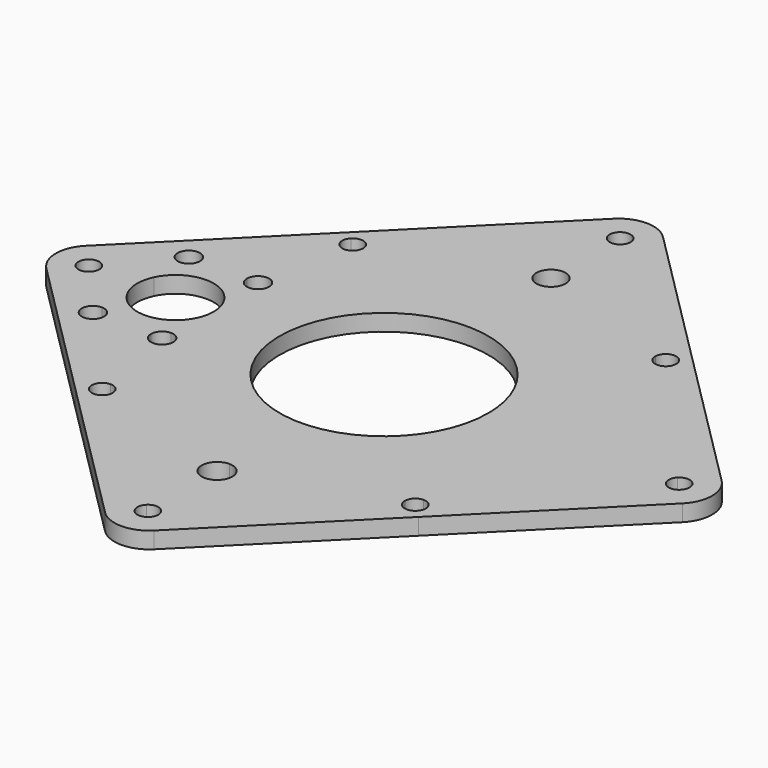
from build123d import *

# Parameters (mm, degrees)
F1_DEPTH = 2.38125
F2_R     = 5
F4_DEPTH = 25
F6_DEPTH = 25


# Not quite as in the source:
# - a feature names something its author has since deleted; it is built from what else it names


with BuildPart() as f1:
    # F0 (on Top) → F1 (new body)
    with BuildSketch(Plane.XY):
        with BuildLine():
            Line((19.9264068712, 22.5), (21.2132034356, 21.2132034356))
            Line((21.2132034356, 21.2132034356), (22.5, 19.9264068712))
            Line((22.5, 19.9264068712), (22.5, 21))
            ThreePointArc((22.5, 21), (21.4393398282, 21.4393398282), (21, 22.5))
            Line((21, 22.5), (19.9264068712, 22.5))
        make_face()
        with BuildLine():
            Line((-41.3657466994, 1.0606601718), (-22.5, 19.9264068712))
            Line((-22.5, 19.9264068712), (-22.5, 21))
            ThreePointArc((-22.5, 21), (-23.8858192988, 21.9259748515), (-23.5606601718, 23.5606601718))
            Line((-23.5606601718, 23.5606601718), (-24.6213203436, 24.6213203436))
            Line((-24.6213203436, 24.6213203436), (-49.2426406871, 0))
            Line((-49.2426406871, 0), (-24.6213203436, -24.6213203436))
            Line((-24.6213203436, -24.6213203436), (-23.5606601718, -23.5606601718))
            ThreePointArc((-23.5606601718, -23.5606601718), (-23.8858192988, -21.9259748515), (-22.5, -21))
            Line((-22.5, -21), (-22.5, -19.9264068712))
            Line((-22.5, -19.9264068712), (-41.3657466994, -1.0606601718))
            ThreePointArc((-41.3657466994, -1.0606601718), (-43.9264068712, 0), (-41.3657466994, 1.0606601718))
        make_face()
        with BuildLine():
            Line((21, -22.5), (19.9264068712, -22.5))
            Line((19.9264068712, -22.5), (1.0606601718, -41.3657466994))
            ThreePointArc((1.0606601718, -41.3657466994), (1.3858192988, -41.8523817226), (1.5, -42.4264068712))
            ThreePointArc((1.5, -42.4264068712), (-0.5740251485, -43.81222617), (-1.0606601718, -41.3657466994))
            Line((-1.0606601718, -41.3657466994), (-19.9264068712, -22.5))
            Line((-19.9264068712, -22.5), (-21, -22.5))
            ThreePointArc((-21, -22.5), (-21.9259748515, -23.8858192988), (-23.5606601718, -23.5606601718))
            Line((-23.5606601718, -23.5606601718), (-24.6213203436, -24.6213203436))
            Line((-24.6213203436, -24.6213203436), (0, -49.2426406871))
            Line((0, -49.2426406871), (24.6213203436, -24.6213203436))
            Line((24.6213203436, -24.6213203436), (23.5606601718, -23.5606601718))
            ThreePointArc((23.5606601718, -23.5606601718), (21.9259748515, -23.8858192988), (21, -22.5))
        make_face()
        with BuildLine():
            Line((22.5, 21), (22.5, 19.9264068712))
            Line((22.5, 19.9264068712), (41.3657466994, 1.0606601718))
            ThreePointArc((41.3657466994, 1.0606601718), (43.0004320197, 1.3858192988), (43.9264068712, 0))
            ThreePointArc((43.9264068712, 0), (43.0004320197, -1.3858192988), (41.3657466994, -1.0606601718))
            Line((41.3657466994, -1.0606601718), (22.5, -19.9264068712))
            Line((22.5, -19.9264068712), (22.5, -21))
            ThreePointArc((22.5, -21), (23.5606601718, -21.4393398282), (24, -22.5))
            ThreePointArc((24, -22.5), (23.8858192988, -23.0740251485), (23.5606601718, -23.5606601718))
            Line((23.5606601718, -23.5606601718), (24.6213203436, -24.6213203436))
            Line((24.6213203436, -24.6213203436), (49.2426406871, 0))
            Line((49.2426406871, 0), (0, 49.2426406871))
            Line((0, 49.2426406871), (-24.6213203436, 24.6213203436))
            Line((-24.6213203436, 24.6213203436), (-23.5606601718, 23.5606601718))
            ThreePointArc((-23.5606601718, 23.5606601718), (-21.9259748515, 23.8858192988), (-21, 22.5))
            Line((-21, 22.5), (-19.9264068712, 22.5))
            Line((-19.9264068712, 22.5), (-1.0606601718, 41.3657466994))
            ThreePointArc((-1.0606601718, 41.3657466994), (-0.5740251485, 43.81222617), (1.5, 42.4264068712))
            ThreePointArc((1.5, 42.4264068712), (1.3858192988, 41.8523817226), (1.0606601718, 41.3657466994))
            Line((1.0606601718, 41.3657466994), (19.9264068712, 22.5))
            Line((19.9264068712, 22.5), (21, 22.5))
            ThreePointArc((21, 22.5), (21.9096815497, 23.8789576234), (23.535365503, 23.585365503))
            ThreePointArc((23.535365503, 23.585365503), (23.8789576234, 23.0903184503), (24, 22.5))
            ThreePointArc((24, 22.5), (23.5606601718, 21.4393398282), (22.5, 21))
        make_face()
        with BuildLine():
            Line((-22.5, -19.9264068712), (-22.5, 19.9264068712))
            Line((-22.5, 19.9264068712), (-41.3657466994, 1.0606601718))
            ThreePointArc((-41.3657466994, 1.0606601718), (-41.0405875724, 0.5740251485), (-40.9264068712, 0))
            ThreePointArc((-40.9264068712, 0), (-41.0405875724, -0.5740251485), (-41.3657466994, -1.0606601718))
            Line((-41.3657466994, -1.0606601718), (-22.5, -19.9264068712))
        make_face()
        with BuildLine():
            Line((-19.9264068712, 22.5), (19.9264068712, 22.5))
            Line((19.9264068712, 22.5), (1.0606601718, 41.3657466994))
            ThreePointArc((1.0606601718, 41.3657466994), (0, 40.9264068712), (-1.0606601718, 41.3657466994))
            Line((-1.0606601718, 41.3657466994), (-19.9264068712, 22.5))
        make_face()
        with BuildLine():
            Line((22.5, 19.9264068712), (22.5, 0))
            Line((22.5, 0), (22.5, -19.9264068712))
            Line((22.5, -19.9264068712), (41.3657466994, -1.0606601718))
            ThreePointArc((41.3657466994, -1.0606601718), (40.9264068712, 0), (41.3657466994, 1.0606601718))
            Line((41.3657466994, 1.0606601718), (22.5, 19.9264068712))
        make_face()
        with BuildLine():
            Line((1.0606601718, -41.3657466994), (19.9264068712, -22.5))
            Line((19.9264068712, -22.5), (-19.9264068712, -22.5))
            Line((-19.9264068712, -22.5), (-1.0606601718, -41.3657466994))
            ThreePointArc((-1.0606601718, -41.3657466994), (0, -40.9264068712), (1.0606601718, -41.3657466994))
        make_face()
        with BuildLine():
            Line((22.5, 0), (15, 0))
            ThreePointArc((15, 0), (-13.8581929877, -5.7402514855), (10.6066017178, 10.6066017178))
            Line((10.6066017178, 10.6066017178), (21.2132034356, 21.2132034356))
            Line((21.2132034356, 21.2132034356), (19.9264068712, 22.5))
            Line((19.9264068712, 22.5), (-19.9264068712, 22.5))
            Line((-19.9264068712, 22.5), (-22.5, 19.9264068712))
            Line((-22.5, 19.9264068712), (-22.5, -19.9264068712))
            Line((-22.5, -19.9264068712), (-19.9264068712, -22.5))
            Line((-19.9264068712, -22.5), (19.9264068712, -22.5))
            Line((19.9264068712, -22.5), (22.5, -19.9264068712))
            Line((22.5, -19.9264068712), (22.5, 0))
        make_face()
        with BuildLine():
            ThreePointArc((10.6066017178, 10.6066017178), (13.8581929877, 5.7402514855), (15, 0))
            Line((15, 0), (22.5, 0))
            Line((22.5, 0), (22.5, 19.9264068712))
            Line((22.5, 19.9264068712), (21.2132034356, 21.2132034356))
            Line((21.2132034356, 21.2132034356), (10.6066017178, 10.6066017178))
        make_face()
        with BuildLine():
            Line((-21, -22.5), (-19.9264068712, -22.5))
            Line((-19.9264068712, -22.5), (-22.5, -19.9264068712))
            Line((-22.5, -19.9264068712), (-22.5, -21))
            ThreePointArc((-22.5, -21), (-21.4393398282, -21.4393398282), (-21, -22.5))
        make_face()
        with BuildLine():
            Line((-22.5, 19.9264068712), (-19.9264068712, 22.5))
            Line((-19.9264068712, 22.5), (-21, 22.5))
            ThreePointArc((-21, 22.5), (-21.4393398282, 21.4393398282), (-22.5, 21))
            Line((-22.5, 21), (-22.5, 19.9264068712))
        make_face()
        with BuildLine():
            Line((22.5, -21), (22.5, -19.9264068712))
            Line((22.5, -19.9264068712), (19.9264068712, -22.5))
            Line((19.9264068712, -22.5), (21, -22.5))
            ThreePointArc((21, -22.5), (21.4393398282, -21.4393398282), (22.5, -21))
        make_face()
    extrude(amount=F1_DEPTH)

    # F2
    f2_edges = [f1.edges().sort_by_distance(p)[0] for p in [
        (0, -49.242641, 1.190625),
        (49.242641, 0, 1.190625),
        (0, 49.242641, 1.190625),
        (-49.242641, 0, 1.190625),
    ]]
    fillet(f2_edges, radius=F2_R)

    # F3 (on face) → F4 (cut)
    with BuildSketch(Plane.XY.offset(2.38125)):
        with BuildLine():
            ThreePointArc((-25, -7.014), (-26.1313708499, -7.4826291501), (-26.6, -8.614))
            Line((-26.6, -8.614), (-25, -8.614))
            Line((-25, -8.614), (-25, -7.014))
        make_face()
        with BuildLine():
            Line((-25, -8.614), (-26.6, -8.614))
            ThreePointArc((-26.6, -8.614), (-25, -10.214), (-23.4, -8.614))
            ThreePointArc((-23.4, -8.614), (-23.8686291501, -7.4826291501), (-25, -7.014))
            Line((-25, -7.014), (-25, -8.614))
        make_face()
        with BuildLine():
            ThreePointArc((-34.948, -7.014), (-36.0793708499, -9.7453708499), (-33.348, -8.614))
            Line((-33.348, -8.614), (-34.948, -8.614))
            Line((-34.948, -8.614), (-34.948, -7.014))
        make_face()
        with BuildLine():
            Line((-34.948, -8.614), (-33.348, -8.614))
            ThreePointArc((-33.348, -8.614), (-33.8166291501, -7.4826291501), (-34.948, -7.014))
            Line((-34.948, -7.014), (-34.948, -8.614))
        make_face()
        with BuildLine():
            ThreePointArc((-34.948, -2.3471949216), (-29.974, -5.5), (-25, -2.3471949216))
            Line((-25, -2.3471949216), (-25, 0))
            Line((-25, 0), (-29.974, 0))
            Line((-29.974, 0), (-34.948, 0))
            Line((-34.948, 0), (-34.948, -2.3471949216))
        make_face()
        with BuildLine():
            Line((-25, 0), (-25, -2.3471949216))
            ThreePointArc((-25, -2.3471949216), (-24.6071107707, -1.2027052839), (-24.474, 0))
            Line((-24.474, 0), (-25, 0))
        make_face()
        with BuildLine():
            ThreePointArc((-34.948, 2.3471949216), (-35.474, 0), (-34.948, -2.3471949216))
            Line((-34.948, -2.3471949216), (-34.948, 0))
            Line((-34.948, 0), (-34.948, 2.3471949216))
        make_face()
        with BuildLine():
            Line((-29.974, 0), (-25, 0))
            Line((-25, 0), (-25, 2.3471949216))
            ThreePointArc((-25, 2.3471949216), (-29.974, 5.5), (-34.948, 2.3471949216))
            Line((-34.948, 2.3471949216), (-34.948, 0))
            Line((-34.948, 0), (-29.974, 0))
        make_face()
        with BuildLine():
            Line((-25, 2.3471949216), (-25, 0))
            Line((-25, 0), (-24.474, 0))
            ThreePointArc((-24.474, 0), (-24.6071107707, 1.2027052839), (-25, 2.3471949216))
        make_face()
        with BuildLine():
            Line((-34.948, 8.614), (-34.948, 7.014))
            ThreePointArc((-34.948, 7.014), (-33.8166291501, 7.4826291501), (-33.348, 8.614))
            Line((-33.348, 8.614), (-34.948, 8.614))
        make_face()
        with BuildLine():
            ThreePointArc((-33.348, 8.614), (-36.0793708499, 9.7453708499), (-34.948, 7.014))
            Line((-34.948, 7.014), (-34.948, 8.614))
            Line((-34.948, 8.614), (-33.348, 8.614))
        make_face()
        with BuildLine():
            ThreePointArc((-26.6, 8.614), (-26.1313708499, 7.4826291501), (-25, 7.014))
            Line((-25, 7.014), (-25, 8.614))
            Line((-25, 8.614), (-26.6, 8.614))
        make_face()
        with BuildLine():
            Line((-25, 8.614), (-25, 7.014))
            ThreePointArc((-25, 7.014), (-23.8686291501, 7.4826291501), (-23.4, 8.614))
            ThreePointArc((-23.4, 8.614), (-25, 10.214), (-26.6, 8.614))
            Line((-26.6, 8.614), (-25, 8.614))
        make_face()
    extrude(amount=-F4_DEPTH, mode=Mode.SUBTRACT)

    # F5 (on face) → F6 (cut)
    with BuildSketch(Plane.XY.offset(2.38125)):
        with BuildLine():
            ThreePointArc((2.2, -30), (1.5556349186, -28.4443650814), (0, -27.8))
            ThreePointArc((0, -27.8), (-1.5556349186, -31.5556349186), (2.2, -30))
        make_face()
        with BuildLine():
            ThreePointArc((2.1, 30), (-1.4849242405, 31.4849242405), (0, 27.9))
            ThreePointArc((0, 27.9), (1.4849242405, 28.5150757595), (2.1, 30))
        make_face()
    extrude(amount=-F6_DEPTH, mode=Mode.SUBTRACT)


solid = f1.part
